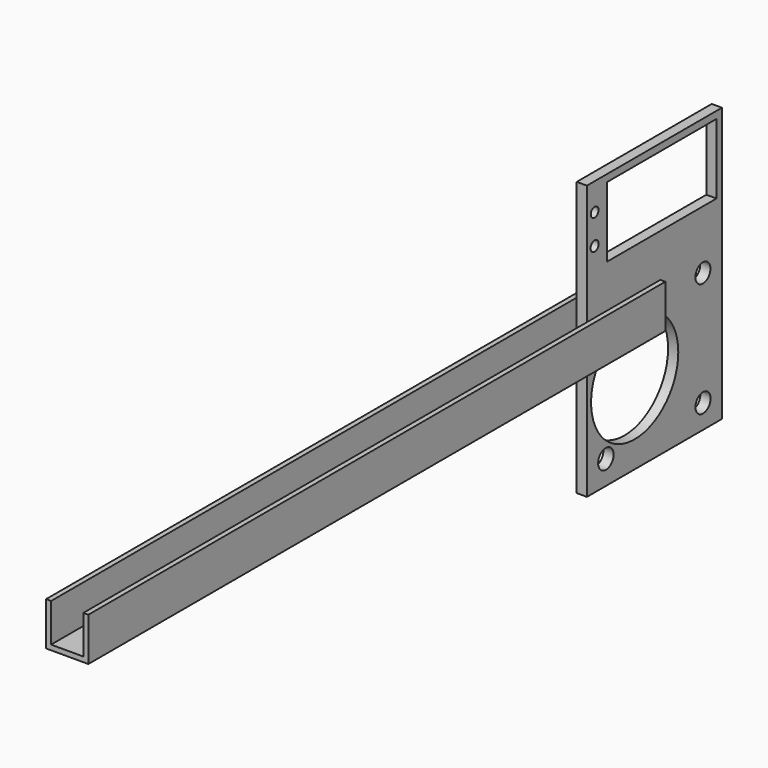
from build123d import *

# Parameters (mm, degrees)
F1_DEPTH = 215.9
F2_W     = 50.5127292126
F2_H     = 82.0375010371
F2_R     = 2.89913405
F2_R_2   = 2.8318920873
F2_R_3   = 2.8588761336
F2_R_4   = 1.5183628154
F2_R_5   = 1.4519166982
F2_R_6   = 2.8173846153
F2_W_2   = 41.0130396485
F2_H_2   = 20.9737662226
F3_DEPTH = 3.06
F5_R     = 16.3147290841
F6_DEPTH = 5


with BuildPart() as f1:
    # F0 (on Front) → F1 (new body)
    with BuildSketch(Plane.XZ):
        Polygon((-4.825, 6.5), (-6.325, 6.5), (-6.325, -6.5), (6.325, -6.5), (6.325, 6.5), (4.825, 6.5), (4.825, -5), (-4.825, -5), align=None)
    extrude(amount=F1_DEPTH)


with BuildPart() as f3:
    # F2 (on Right) → F3 (new body)
    with BuildSketch(Plane.YZ):
        with Locations((0.0250553712, 0.0057928264)):
            Rectangle(F2_W, F2_H)
        with Locations((-18.1433722998, -33.8706020266)):
            Circle(F2_R, mode=Mode.SUBTRACT)
        with Locations((18.2029870339, -33.8714673854)):
            Circle(F2_R_2, mode=Mode.SUBTRACT)
        with Locations((-18.0760649964, 0.4261299481)):
            Circle(F2_R_3, mode=Mode.SUBTRACT)
        with Locations((-22.3539447378, 23.9319726942)):
            Circle(F2_R_4, mode=Mode.SUBTRACT)
        with Locations((-22.3546241195, 32.8359914765)):
            Circle(F2_R_5, mode=Mode.SUBTRACT)
        with Locations((18.1693327613, 0.3677118686)):
            Circle(F2_R_6, mode=Mode.SUBTRACT)
        with Locations((2.7500502765, 28.4059746191)):
            Rectangle(F2_W_2, F2_H_2, mode=Mode.SUBTRACT)
    extrude(amount=F3_DEPTH)

    # F5 (on face) → F6 (cut)
    with BuildSketch(Plane.YZ.offset(3.06)):
        with Locations((-7.363283649, -16.781862238)):
            Circle(F5_R)
    extrude(amount=-F6_DEPTH, mode=Mode.SUBTRACT)


solid = Compound([f1.part, f3.part])
